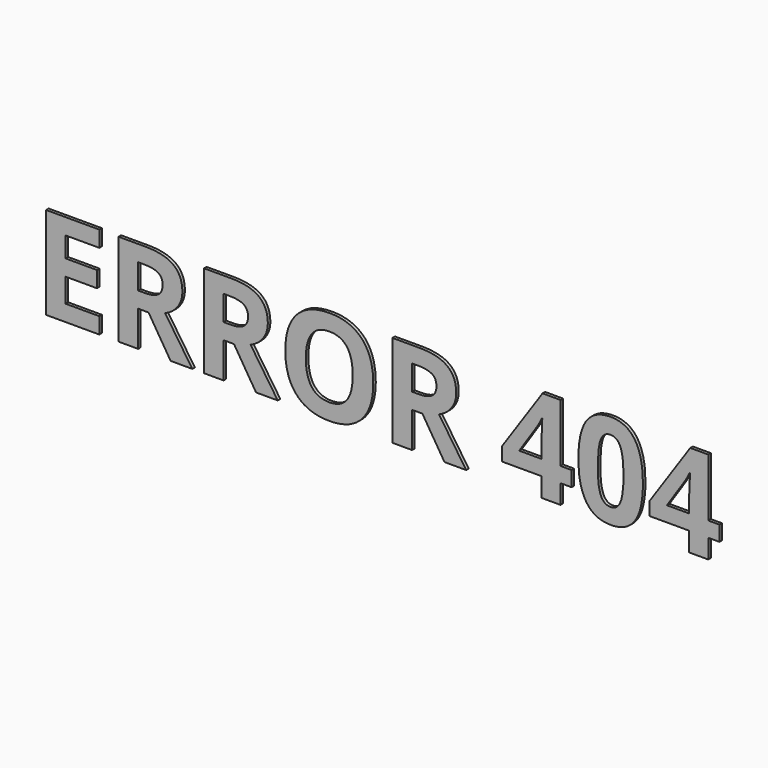
from build123d import *

# Parameters (mm, degrees)
F0_TEXT_SIZE = 103.6646124985
F1_DEPTH     = 2.54


# Not quite as in the source:
# - Text() gives the source's letters only with a copy of the font that has no kerning and outlines rounded to 1/6400 em; it was checked with that copy


with BuildPart() as f1:
    # F0 (on Front) → F1 (new body)
    with BuildSketch(Plane.XZ):
        with Locations((-277.707778326, -37.3192604994)):
            Text('ERROR 404', F0_TEXT_SIZE, font='Open Sans', font_style=FontStyle.BOLD, text_align=(TextAlign.LEFT, TextAlign.BOTTOM))
    extrude(amount=F1_DEPTH)


solid = f1.part
